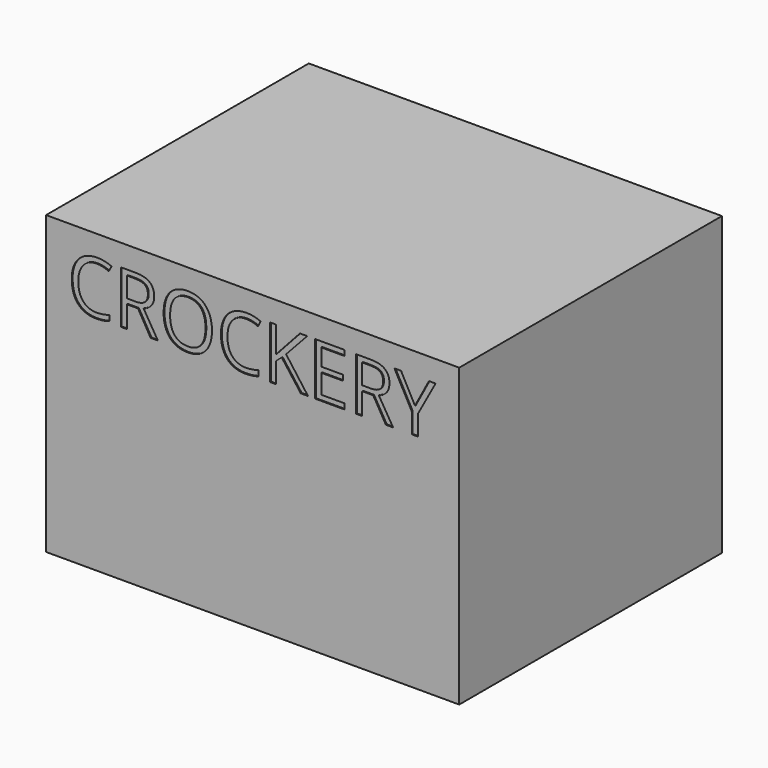
from build123d import *

# Parameters (mm, degrees)
F0_W         = 390
F0_H         = 310
F1_DEPTH     = 280
F2_TEXT_SIZE = 69.4444444444
F3_DEPTH     = 1


# Not quite as in the source:
# - Text() gives the source's letters only with a copy of the font that has no kerning and outlines rounded to 1/6400 em; it was checked with that copy


with BuildPart() as f1:
    # F0 (on Top) → F1 (new body)
    with BuildSketch(Plane.XY):
        Rectangle(F0_W, F0_H)
    extrude(amount=F1_DEPTH)

    # F2 (on face) → F3 (cut)
    with BuildSketch(Plane.XZ.offset(155)):
        with Locations((-175, 210)):
            Text('CROCKERY', F2_TEXT_SIZE, font='Open Sans', text_align=(TextAlign.LEFT, TextAlign.BOTTOM))
    extrude(amount=-F3_DEPTH, mode=Mode.SUBTRACT)


solid = f1.part
